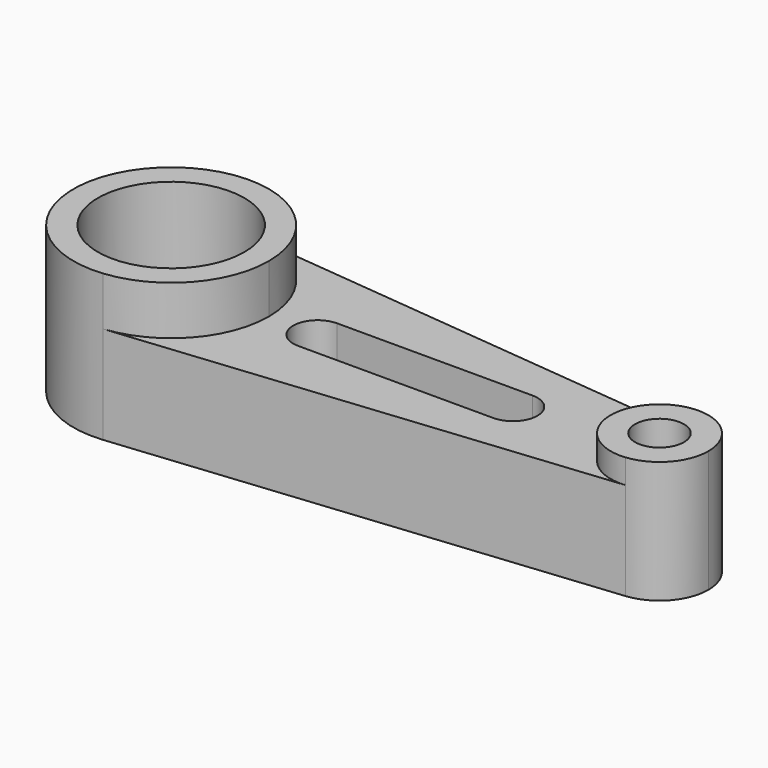
from build123d import *
from build123d import SkipClean  # not in build123d's __all__

# Parameters (mm, degrees)
F0_R     = 19.05
F0_R_2   = 6.35
F1_DEPTH = 38.1
F2_DEPTH = 12.7
F3_DEPTH = 6.35


with BuildPart() as f1:
    # F0 (on Top) → F1 (new body)
    with BuildSketch(Plane.XY):
        with BuildLine():
            ThreePointArc((-59.2360458782, -25.2726809025), (-42.9389017209, -17.0388379885), (-36.3760458782, 0))
            ThreePointArc((-36.3760458782, 0), (-42.9389017209, 17.0388379885), (-59.2360458782, 25.2726809025))
            ThreePointArc((-59.2360458782, 25.2726809025), (-87.1760458782, 0), (-59.2360458782, -25.2726809025))
        make_face()
        with Locations((-61.7760458782, 0)):
            Circle(F0_R, mode=Mode.SUBTRACT)
        with BuildLine():
            ThreePointArc((-59.2360458782, 25.2726809025), (-42.9389017209, 17.0388379885), (-36.3760458782, 0))
            ThreePointArc((-36.3760458782, 0), (-42.9389017209, -17.0388379885), (-59.2360458782, -25.2726809025))
            Line((-59.2360458782, -25.2726809025), (66.4939541218, -12.6363404513))
            ThreePointArc((66.4939541218, -12.6363404513), (52.5239541218, 0), (66.4939541218, 12.6363404513))
            Line((66.4939541218, 12.6363404513), (-59.2360458782, 25.2726809025))
        make_face()
        with BuildLine():
            ThreePointArc((-23.6760458782, -6.35), (-30.0260458782, 0), (-23.6760458782, 6.35))
            Line((-23.6760458782, 6.35), (27.1239541218, 6.35))
            ThreePointArc((27.1239541218, 6.35), (33.4739541218, 0), (27.1239541218, -6.35))
            Line((27.1239541218, -6.35), (-23.6760458782, -6.35))
        make_face(mode=Mode.SUBTRACT)
        with BuildLine():
            ThreePointArc((77.9239541218, 0), (74.6425262005, 8.5194189943), (66.4939541218, 12.6363404513))
            ThreePointArc((66.4939541218, 12.6363404513), (52.5239541218, 0), (66.4939541218, -12.6363404513))
            ThreePointArc((66.4939541218, -12.6363404513), (74.6425262005, -8.5194189943), (77.9239541218, 0))
        make_face()
        with Locations((65.2239541218, 0)):
            Circle(F0_R_2, mode=Mode.SUBTRACT)
    extrude(amount=-F1_DEPTH)

    # F0 (on Top) → F2 (cut)
    with BuildSketch(Plane.XY):
        with BuildLine():
            ThreePointArc((-59.2360458782, 25.2726809025), (-42.9389017209, 17.0388379885), (-36.3760458782, 0))
            ThreePointArc((-36.3760458782, 0), (-42.9389017209, -17.0388379885), (-59.2360458782, -25.2726809025))
            Line((-59.2360458782, -25.2726809025), (66.4939541218, -12.6363404513))
            ThreePointArc((66.4939541218, -12.6363404513), (52.5239541218, 0), (66.4939541218, 12.6363404513))
            Line((66.4939541218, 12.6363404513), (-59.2360458782, 25.2726809025))
        make_face()
        with BuildLine():
            ThreePointArc((-23.6760458782, -6.35), (-30.0260458782, 0), (-23.6760458782, 6.35))
            Line((-23.6760458782, 6.35), (27.1239541218, 6.35))
            ThreePointArc((27.1239541218, 6.35), (33.4739541218, 0), (27.1239541218, -6.35))
            Line((27.1239541218, -6.35), (-23.6760458782, -6.35))
        make_face(mode=Mode.SUBTRACT)
    with SkipClean():  # cleaning this boolean's faces spoils the solid; the shape is the same uncleaned
        extrude(amount=-F2_DEPTH, mode=Mode.SUBTRACT)

    # F3 (cut): a face of the model
    f3_faces = [f1.faces().sort_by_distance(p)[0] for p in [
        (77.564743877, 0, 0),
    ]]
    extrude(f3_faces, amount=-F3_DEPTH, mode=Mode.SUBTRACT)


solid = f1.part
